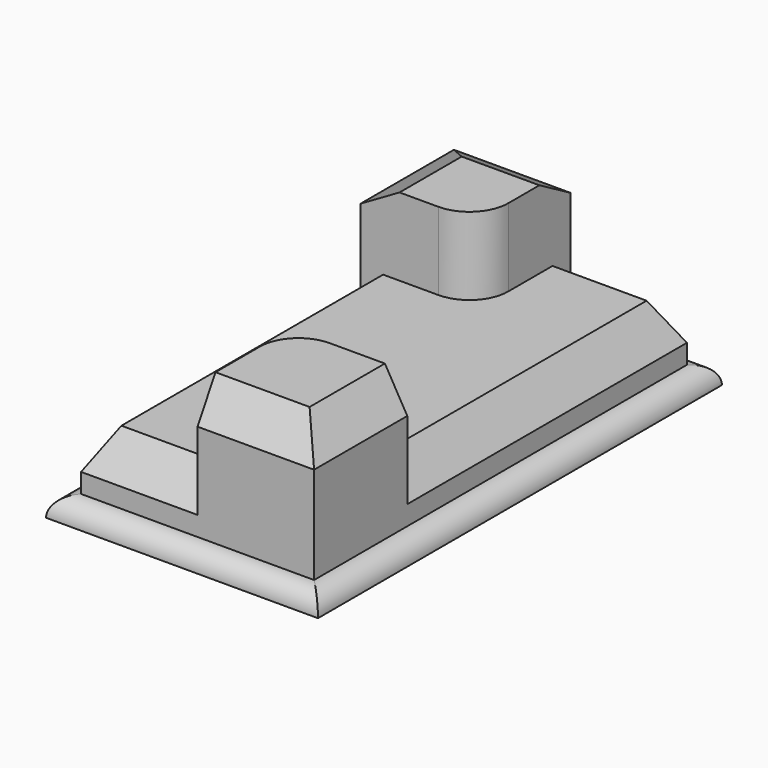
from build123d import *

# Parameters (mm, degrees)
F0_W        = 88.9
F0_H        = 165.1
F1_DEPTH    = 6.35
F2_DEPTH    = 25.4
F3_DEPTH    = 50.8
F4_C1_SIZE2 = 12.7
F4_C1_SIZE  = 7.3323484187
F4_C2_SIZE2 = 7.3323484187
F4_C2_SIZE  = 12.7
F4_C3_SIZE2 = 12.7
F4_C3_SIZE  = 7.3323484187
F4_C4_SIZE2 = 7.3323484187
F4_C4_SIZE  = 12.7
F4_C5_SIZE2 = 12.7
F4_C5_SIZE  = 7.3323484187
F4_C6_SIZE2 = 7.3323484187
F4_C6_SIZE  = 12.7
F4_C7_SIZE2 = 12.7
F4_C7_SIZE  = 7.3323484187
F4_C8_SIZE2 = 12.7
F4_C8_SIZE  = 7.3323484187
F5_R        = 6.34999


# Not quite as in the source:
# - a fillet or chamfer is up to 0.001 mm smaller than in the source, because OpenCascade refuses the exact size


with BuildPart() as f1:
    # F0 (on Top) → F1 (new body)
    with BuildSketch(Plane.XY):
        Rectangle(F0_W, F0_H)
        Polygon((0, 76.2), (38.1, 76.2), (38.1, -38.1), (38.1, -76.2), (0, -76.2), (-38.1, -76.2), (-38.1, 38.1), (-38.1, 76.2), align=None, mode=Mode.SUBTRACT)
    extrude(amount=F1_DEPTH)

    # F0 (on Top) → F2 (join)
    with BuildSketch(Plane.XY):
        with BuildLine():
            Line((38.1, -38.1), (38.1, 76.2))
            Line((38.1, 76.2), (0, 76.2))
            Line((0, 76.2), (0, 50.8))
            ThreePointArc((0, 50.8), (-3.7197438789, 41.8197438789), (-12.7, 38.1))
            Line((-12.7, 38.1), (-38.1, 38.1))
            Line((-38.1, 38.1), (-38.1, -76.2))
            Line((-38.1, -76.2), (0, -76.2))
            Line((0, -76.2), (0, -50.8))
            ThreePointArc((0, -50.8), (3.7197438789, -41.8197438789), (12.7, -38.1))
            Line((12.7, -38.1), (38.1, -38.1))
        make_face()
    extrude(amount=F2_DEPTH)

    # F0 (on Top) → F3 (join)
    with BuildSketch(Plane.XY):
        with BuildLine():
            Line((0, 50.8), (0, 76.2))
            Line((0, 76.2), (-38.1, 76.2))
            Line((-38.1, 76.2), (-38.1, 38.1))
            Line((-38.1, 38.1), (-12.7, 38.1))
            ThreePointArc((-12.7, 38.1), (-3.7197438789, 41.8197438789), (0, 50.8))
        make_face()
        with BuildLine():
            Line((38.1, -76.2), (38.1, -38.1))
            Line((38.1, -38.1), (12.7, -38.1))
            ThreePointArc((12.7, -38.1), (3.7197438789, -41.8197438789), (0, -50.8))
            Line((0, -50.8), (0, -76.2))
            Line((0, -76.2), (38.1, -76.2))
        make_face()
    extrude(amount=F3_DEPTH)

    # F4: chamfer of 12.7 x 7.3323484187 on 8 edges, made by hand

    # F4_c1
    f4_c1_edges = [f1.edges().sort_by_distance(p)[0] for p in [
        (-38.1, 57.15, 50.8),
    ]]
    f4_c1_side = f1.faces().sort_by_distance((-38.1, 57.15, 50.6533530316))[0]
    chamfer(f4_c1_edges, length=F4_C1_SIZE, length2=F4_C1_SIZE2, reference=f4_c1_side)

    # F4_c2
    f4_c2_edges = [f1.edges().sort_by_distance(p)[0] for p in [
        (-38.1, -19.05, 25.4),
    ]]
    f4_c2_side = f1.faces().sort_by_distance((-38.1, -19.05, 25.2533530316))[0]
    chamfer(f4_c2_edges, length=F4_C2_SIZE, length2=F4_C2_SIZE2, reference=f4_c2_side)

    # F4_c3
    f4_c3_edges = [f1.edges().sort_by_distance(p)[0] for p in [
        (38.1, 19.05, 25.4),
    ]]
    f4_c3_side = f1.faces().sort_by_distance((37.9533530316, 19.05, 25.4))[0]
    chamfer(f4_c3_edges, length=F4_C3_SIZE, length2=F4_C3_SIZE2, reference=f4_c3_side)

    # F4_c4
    f4_c4_edges = [f1.edges().sort_by_distance(p)[0] for p in [
        (15.3838257906, 76.2, 25.4),
    ]]
    f4_c4_side = f1.faces().sort_by_distance((15.3838257906, 76.2, 25.2533530316))[0]
    chamfer(f4_c4_edges, length=F4_C4_SIZE, length2=F4_C4_SIZE2, reference=f4_c4_side)

    # F4_c5
    f4_c5_edges = [f1.edges().sort_by_distance(p)[0] for p in [
        (-15.3838257906, -76.2, 25.4),
    ]]
    f4_c5_side = f1.faces().sort_by_distance((-15.3838257906, -76.0533530316, 25.4))[0]
    chamfer(f4_c5_edges, length=F4_C5_SIZE, length2=F4_C5_SIZE2, reference=f4_c5_side)

    # F4_c6
    f4_c6_edges = [f1.edges().sort_by_distance(p)[0] for p in [
        (19.05, -76.2, 50.8),
    ]]
    f4_c6_side = f1.faces().sort_by_distance((19.05, -76.2, 50.6533530316))[0]
    chamfer(f4_c6_edges, length=F4_C6_SIZE, length2=F4_C6_SIZE2, reference=f4_c6_side)

    # F4_c7
    f4_c7_edges = [f1.edges().sort_by_distance(p)[0] for p in [
        (38.1, -53.4838257906, 50.8),
    ]]
    f4_c7_side = f1.faces().sort_by_distance((37.9533530316, -53.4838257906, 50.8))[0]
    chamfer(f4_c7_edges, length=F4_C7_SIZE, length2=F4_C7_SIZE2, reference=f4_c7_side)

    # F4_c8
    f4_c8_edges = [f1.edges().sort_by_distance(p)[0] for p in [
        (-12.7, 76.2, 50.8),
    ]]
    f4_c8_side = f1.faces().sort_by_distance((-12.7, 76.2, 50.6533530316))[0]
    chamfer(f4_c8_edges, length=F4_C8_SIZE, length2=F4_C8_SIZE2, reference=f4_c8_side)

    # F5 (radius 6.35 in the source; OpenCascade refuses exactly that, so slightly less here)
    f5_edges = [f1.edges().sort_by_distance(p)[0] for p in [
        (44.45, 0, 6.35),
        (0, 82.55, 6.35),
        (0, -82.55, 6.35),
        (-44.45, 0, 6.35),
    ]]
    fillet(f5_edges, radius=F5_R)


solid = f1.part
